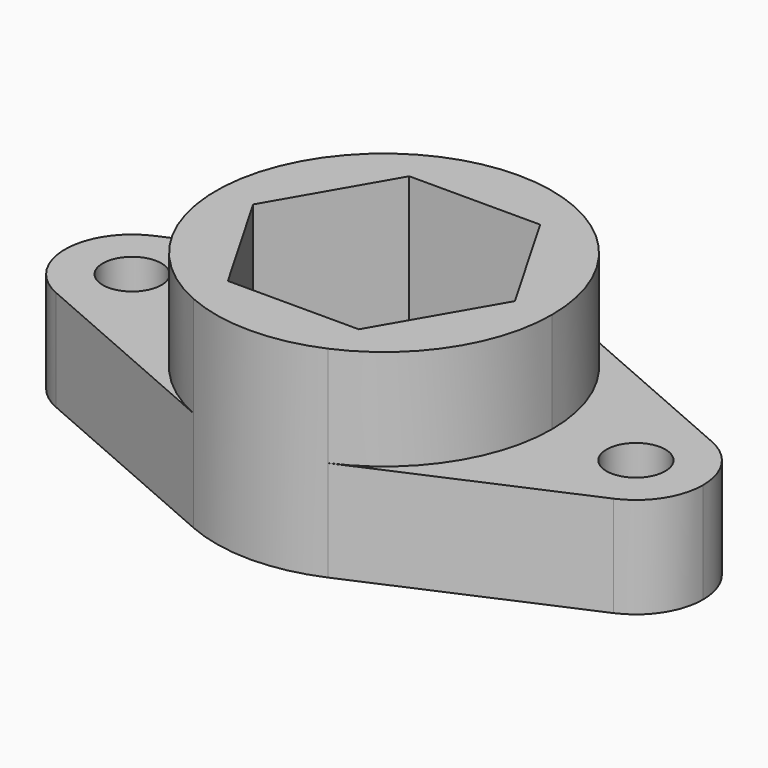
from build123d import *

# Parameters (mm, degrees)
F1_DEPTH = 11
F2_DEPTH = 5
F3_DEPTH = 1
F4_DEPTH = 5
F5_D     = 3.5


with BuildPart() as f1:
    # F0 (on Top) → F1 (new body)
    with BuildSketch(Plane.XY):
        with BuildLine():
            Line((-3.897114, 6.75), (-2.945942, 6.75))
            Line((-2.945942, 6.75), (-4, 9.165151))
            ThreePointArc((-4, 9.165151), (-10, 0), (-4, -9.165151))
            Line((-4, -9.165151), (-2.945942, -6.75))
            Line((-2.945942, -6.75), (-3.897114, -6.75))
            Line((-3.897114, -6.75), (-7.794229, 0))
            Line((-7.794229, 0), (-3.897114, 6.75))
        make_face()
        with BuildLine():
            Line((-2.945942, 6.75), (2.945942, 6.75))
            Line((2.945942, 6.75), (4, 9.165151))
            ThreePointArc((4, 9.165151), (0, 10), (-4, 9.165151))
            Line((-4, 9.165151), (-2.945942, 6.75))
        make_face()
        with BuildLine():
            Line((4, 9.165151), (2.945942, 6.75))
            Line((2.945942, 6.75), (3.897114, 6.75))
            Line((3.897114, 6.75), (7.794229, 0))
            Line((7.794229, 0), (3.897114, -6.75))
            Line((3.897114, -6.75), (2.945942, -6.75))
            Line((2.945942, -6.75), (4, -9.165151))
            ThreePointArc((4, -9.165151), (8.3666, -5.477226), (10, 0))
            ThreePointArc((10, 0), (8.3666, 5.477226), (4, 9.165151))
        make_face()
        with BuildLine():
            Line((4, -9.165151), (2.945942, -6.75))
            Line((2.945942, -6.75), (-2.945942, -6.75))
            Line((-2.945942, -6.75), (-4, -9.165151))
            ThreePointArc((-4, -9.165151), (0, -10), (4, -9.165151))
        make_face()
    extrude(amount=F1_DEPTH)

    # F0 (on Top) → F2 (join)
    with BuildSketch(Plane.XY):
        with BuildLine():
            ThreePointArc((-4, -9.165151), (-10, 0), (-4, 9.165151))
            Line((-4, 9.165151), (-16.6, 3.666061))
            ThreePointArc((-16.6, 3.666061), (-12.80911, 3.34664), (-11, 0))
            ThreePointArc((-11, 0), (-12.80911, -3.34664), (-16.6, -3.666061))
            Line((-16.6, -3.666061), (-4, -9.165151))
        make_face()
        with BuildLine():
            ThreePointArc((-11, 0), (-12.80911, 3.34664), (-16.6, 3.666061))
            Line((-16.6, 3.666061), (-15.7, 1.603901))
            ThreePointArc((-15.7, 1.603901), (-14.041486, 1.464155), (-13.25, 0))
            ThreePointArc((-13.25, 0), (-14.041486, -1.464155), (-15.7, -1.603901))
            Line((-15.7, -1.603901), (-16.6, -3.666061))
            ThreePointArc((-16.6, -3.666061), (-12.80911, -3.34664), (-11, 0))
        make_face()
        with BuildLine():
            Line((-15.7, 1.603901), (-16.6, 3.666061))
            ThreePointArc((-16.6, 3.666061), (-19, 0), (-16.6, -3.666061))
            Line((-16.6, -3.666061), (-15.7, -1.603901))
            ThreePointArc((-15.7, -1.603901), (-16.75, 0), (-15.7, 1.603901))
        make_face()
        with BuildLine():
            Line((16.6, 3.666061), (4, 9.165151))
            ThreePointArc((4, 9.165151), (8.3666, 5.477226), (10, 0))
            ThreePointArc((10, 0), (8.3666, -5.477226), (4, -9.165151))
            Line((4, -9.165151), (16.6, -3.666061))
            ThreePointArc((16.6, -3.666061), (11, 0), (16.6, 3.666061))
        make_face()
        with BuildLine():
            Line((15.7, 1.603901), (16.6, 3.666061))
            ThreePointArc((16.6, 3.666061), (11, 0), (16.6, -3.666061))
            Line((16.6, -3.666061), (15.7, -1.603901))
            ThreePointArc((15.7, -1.603901), (13.25, 0), (15.7, 1.603901))
        make_face()
        with BuildLine():
            ThreePointArc((19, 0), (18.34664, 2.19089), (16.6, 3.666061))
            Line((16.6, 3.666061), (15.7, 1.603901))
            ThreePointArc((15.7, 1.603901), (16.464155, 0.958514), (16.75, 0))
            ThreePointArc((16.75, 0), (16.464155, -0.958514), (15.7, -1.603901))
            Line((15.7, -1.603901), (16.6, -3.666061))
            ThreePointArc((16.6, -3.666061), (18.34664, -2.19089), (19, 0))
        make_face()
    extrude(amount=F2_DEPTH)

    # F0 (on Top) → F3 (join)
    with BuildSketch(Plane.XY):
        with BuildLine():
            Line((-15.7, 1.603901), (-16.6, 3.666061))
            ThreePointArc((-16.6, 3.666061), (-19, 0), (-16.6, -3.666061))
            Line((-16.6, -3.666061), (-15.7, -1.603901))
            ThreePointArc((-15.7, -1.603901), (-16.75, 0), (-15.7, 1.603901))
        make_face()
        with BuildLine():
            ThreePointArc((-11, 0), (-12.80911, 3.34664), (-16.6, 3.666061))
            Line((-16.6, 3.666061), (-15.7, 1.603901))
            ThreePointArc((-15.7, 1.603901), (-14.041486, 1.464155), (-13.25, 0))
            ThreePointArc((-13.25, 0), (-14.041486, -1.464155), (-15.7, -1.603901))
            Line((-15.7, -1.603901), (-16.6, -3.666061))
            ThreePointArc((-16.6, -3.666061), (-12.80911, -3.34664), (-11, 0))
        make_face()
        with BuildLine():
            ThreePointArc((-4, -9.165151), (-10, 0), (-4, 9.165151))
            Line((-4, 9.165151), (-16.6, 3.666061))
            ThreePointArc((-16.6, 3.666061), (-12.80911, 3.34664), (-11, 0))
            ThreePointArc((-11, 0), (-12.80911, -3.34664), (-16.6, -3.666061))
            Line((-16.6, -3.666061), (-4, -9.165151))
        make_face()
        with BuildLine():
            Line((-3.897114, 6.75), (-2.945942, 6.75))
            Line((-2.945942, 6.75), (-4, 9.165151))
            ThreePointArc((-4, 9.165151), (-10, 0), (-4, -9.165151))
            Line((-4, -9.165151), (-2.945942, -6.75))
            Line((-2.945942, -6.75), (-3.897114, -6.75))
            Line((-3.897114, -6.75), (-7.794229, 0))
            Line((-7.794229, 0), (-3.897114, 6.75))
        make_face()
        with BuildLine():
            Line((4, -9.165151), (2.945942, -6.75))
            Line((2.945942, -6.75), (-2.945942, -6.75))
            Line((-2.945942, -6.75), (-4, -9.165151))
            ThreePointArc((-4, -9.165151), (0, -10), (4, -9.165151))
        make_face()
        with BuildLine():
            Line((-2.945942, 6.75), (2.945942, 6.75))
            Line((2.945942, 6.75), (4, 9.165151))
            ThreePointArc((4, 9.165151), (0, 10), (-4, 9.165151))
            Line((-4, 9.165151), (-2.945942, 6.75))
        make_face()
        with BuildLine():
            Line((4, 9.165151), (2.945942, 6.75))
            Line((2.945942, 6.75), (3.897114, 6.75))
            Line((3.897114, 6.75), (7.794229, 0))
            Line((7.794229, 0), (3.897114, -6.75))
            Line((3.897114, -6.75), (2.945942, -6.75))
            Line((2.945942, -6.75), (4, -9.165151))
            ThreePointArc((4, -9.165151), (8.3666, -5.477226), (10, 0))
            ThreePointArc((10, 0), (8.3666, 5.477226), (4, 9.165151))
        make_face()
        with BuildLine():
            Line((16.6, 3.666061), (4, 9.165151))
            ThreePointArc((4, 9.165151), (8.3666, 5.477226), (10, 0))
            ThreePointArc((10, 0), (8.3666, -5.477226), (4, -9.165151))
            Line((4, -9.165151), (16.6, -3.666061))
            ThreePointArc((16.6, -3.666061), (11, 0), (16.6, 3.666061))
        make_face()
        with BuildLine():
            Line((15.7, 1.603901), (16.6, 3.666061))
            ThreePointArc((16.6, 3.666061), (11, 0), (16.6, -3.666061))
            Line((16.6, -3.666061), (15.7, -1.603901))
            ThreePointArc((15.7, -1.603901), (13.25, 0), (15.7, 1.603901))
        make_face()
        with BuildLine():
            ThreePointArc((19, 0), (18.34664, 2.19089), (16.6, 3.666061))
            Line((16.6, 3.666061), (15.7, 1.603901))
            ThreePointArc((15.7, 1.603901), (16.464155, 0.958514), (16.75, 0))
            ThreePointArc((16.75, 0), (16.464155, -0.958514), (15.7, -1.603901))
            Line((15.7, -1.603901), (16.6, -3.666061))
            ThreePointArc((16.6, -3.666061), (18.34664, -2.19089), (19, 0))
        make_face()
        with BuildLine():
            ThreePointArc((-1.8, -4.124318), (-4.5, 0), (-1.8, 4.124318))
            Line((-1.8, 4.124318), (-2.945942, 6.75))
            Line((-2.945942, 6.75), (-3.897114, 6.75))
            Line((-3.897114, 6.75), (-7.794229, 0))
            Line((-7.794229, 0), (-3.897114, -6.75))
            Line((-3.897114, -6.75), (-2.945942, -6.75))
            Line((-2.945942, -6.75), (-1.8, -4.124318))
        make_face()
        with BuildLine():
            Line((2.945942, -6.75), (1.8, -4.124318))
            ThreePointArc((1.8, -4.124318), (0, -4.5), (-1.8, -4.124318))
            Line((-1.8, -4.124318), (-2.945942, -6.75))
            Line((-2.945942, -6.75), (2.945942, -6.75))
        make_face()
        with BuildLine():
            ThreePointArc((1.8, 4.124318), (3.76497, 2.464752), (4.5, 0))
            ThreePointArc((4.5, 0), (3.76497, -2.464752), (1.8, -4.124318))
            Line((1.8, -4.124318), (2.945942, -6.75))
            Line((2.945942, -6.75), (3.897114, -6.75))
            Line((3.897114, -6.75), (7.794229, 0))
            Line((7.794229, 0), (3.897114, 6.75))
            Line((3.897114, 6.75), (2.945942, 6.75))
            Line((2.945942, 6.75), (1.8, 4.124318))
        make_face()
        with BuildLine():
            ThreePointArc((-1.8, 4.124318), (0, 4.5), (1.8, 4.124318))
            Line((1.8, 4.124318), (2.945942, 6.75))
            Line((2.945942, 6.75), (-2.945942, 6.75))
            Line((-2.945942, 6.75), (-1.8, 4.124318))
        make_face()
    extrude(amount=-F3_DEPTH)

    # F0 (on Top) → F4 (join)
    with BuildSketch(Plane.XY):
        with BuildLine():
            Line((15, 0), (15.7, 1.603901))
            ThreePointArc((15.7, 1.603901), (13.25, 0), (15.7, -1.603901))
            Line((15.7, -1.603901), (15, 0))
        make_face()
        with BuildLine():
            ThreePointArc((16.75, 0), (16.464155, 0.958514), (15.7, 1.603901))
            Line((15.7, 1.603901), (15, 0))
            Line((15, 0), (15.7, -1.603901))
            ThreePointArc((15.7, -1.603901), (16.464155, -0.958514), (16.75, 0))
        make_face()
        with BuildLine():
            ThreePointArc((-13.25, 0), (-14.041486, 1.464155), (-15.7, 1.603901))
            Line((-15.7, 1.603901), (-15, 0))
            Line((-15, 0), (-15.7, -1.603901))
            ThreePointArc((-15.7, -1.603901), (-14.041486, -1.464155), (-13.25, 0))
        make_face()
        with BuildLine():
            Line((-15, 0), (-15.7, 1.603901))
            ThreePointArc((-15.7, 1.603901), (-16.75, 0), (-15.7, -1.603901))
            Line((-15.7, -1.603901), (-15, 0))
        make_face()
    extrude(amount=F4_DEPTH)

    # F5 (through all)
    with Locations(Plane(origin=(0, 0, 0), x_dir=(1, 0, 0), z_dir=(0, 0, -1))):
        with Locations((15, 0), (-15, 0)):
            Hole(F5_D / 2)


solid = f1.part
